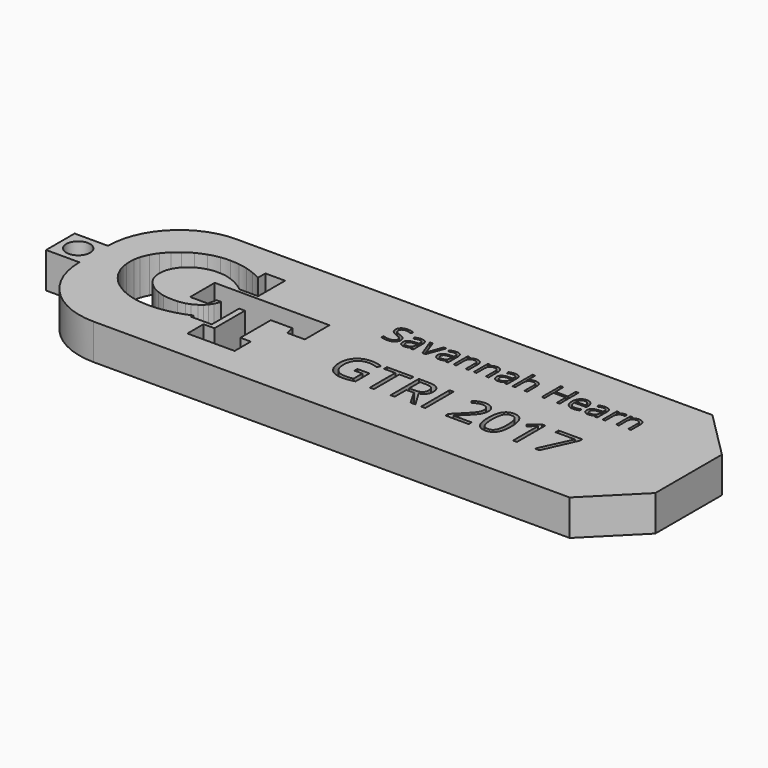
from build123d import *

# Parameters (mm, degrees)
F0_W         = 63.5
F0_H         = 19.05
F1_DEPTH     = 3.81
F3_DEPTH     = 3.81
F4_SIZE      = 5.08
F5_SIZE      = 5.08
F6_R         = 7.62
F7_R         = 7.62
F8_TEXT_SIZE = 3.5277777778
F10_DEPTH    = 1.524
F9_TEXT_SIZE = 5.2916666667
F11_DEPTH    = 1.524
F12_W        = 3.81
F12_H        = 3.81
F13_DEPTH    = 3.556
F15_D        = 2.54


# Not quite as in the source:
# - Text() gives the source's letters only with a copy of the font that has no kerning and outlines rounded to 1/6400 em; it was checked with that copy


with BuildPart() as f1:
    # F0 (on Top) → F1 (new body)
    with BuildSketch(Plane.XY):
        with Locations((31.75, -38.8746707218)):
            Rectangle(F0_W, F0_H)
    extrude(amount=F1_DEPTH)

    # F2 (on face) → F3 (cut)
    with BuildSketch(Plane.XY.offset(3.81)):
        with BuildLine():
            ThreePointArc((9.6262898296, -32.6765216887), (9.1345656228, -32.6782186949), (8.6470656097, -32.7425561845))
            ThreePointArc((8.6470656097, -32.7425561845), (8.0416604213, -32.8459942993), (7.4538225308, -33.0239310861))
            ThreePointArc((7.4538225308, -33.0239310861), (6.9355950201, -33.2250870831), (6.4325318672, -33.4616266191))
            ThreePointArc((6.4325318672, -33.4616266191), (5.9624118467, -33.7301717613), (5.5258763023, -34.0504311025))
            ThreePointArc((5.5258763023, -34.0504311025), (5.1852816432, -34.3165591196), (4.8669776879, -34.6089825034))
            ThreePointArc((4.8669776879, -34.6089825034), (4.5097063038, -34.9592664571), (4.1853138246, -35.3402011096))
            ThreePointArc((4.1853138246, -35.3402011096), (3.942059585, -35.6919738597), (3.7296244409, -36.0631719232))
            ThreePointArc((3.7296244409, -36.0631719232), (3.531707517, -36.4810877637), (3.3790939488, -36.9175896049))
            ThreePointArc((3.3790939488, -36.9175896049), (3.2938530275, -37.2302091826), (3.2438719645, -37.5503636897))
            ThreePointArc((3.2438719645, -37.5503636897), (3.2157331662, -38.0625072867), (3.2438719645, -38.5746508837))
            ThreePointArc((3.2438719645, -38.5746508837), (3.2872944597, -38.8672702316), (3.3429092728, -39.1578190029))
            ThreePointArc((3.3429092728, -39.1578190029), (3.3975529318, -39.3800627955), (3.4688711166, -39.597529918))
            ThreePointArc((3.4688711166, -39.597529918), (3.5952100841, -39.8924262154), (3.7296244409, -40.1837304235))
            ThreePointArc((3.7296244409, -40.1837304235), (3.8898334232, -40.4674932421), (4.0712854825, -40.7381653786))
            ThreePointArc((4.0712854825, -40.7381653786), (4.2164038702, -40.9343188623), (4.3698656373, -41.1240160465))
            ThreePointArc((4.3698656373, -41.1240160465), (4.4748950547, -41.2464015486), (4.5850998722, -41.3641482592))
            ThreePointArc((4.5850998722, -41.3641482592), (4.7484852476, -41.5319231994), (4.9246759154, -41.6861958802))
            ThreePointArc((4.9246759154, -41.6861958802), (5.085215868, -41.8163599874), (5.2489168011, -41.942525655))
            ThreePointArc((5.2489168011, -41.942525655), (5.3654646363, -42.0288014147), (5.4855244234, -42.110119015))
            ThreePointArc((5.4855244234, -42.110119015), (5.6214336133, -42.2028707503), (5.7604718022, -42.2908626497))
            ThreePointArc((5.7604718022, -42.2908626497), (5.8741145853, -42.3605784939), (5.9905075468, -42.4255989492))
            ThreePointArc((5.9905075468, -42.4255989492), (6.2169238827, -42.5464367765), (6.4516742714, -42.6501594484))
            ThreePointArc((6.4516742714, -42.6501594484), (6.7163385506, -42.7569305989), (6.9818515331, -42.8615733981))
            ThreePointArc((6.9818515331, -42.8615733981), (7.2850539518, -42.9552044529), (7.5919940136, -43.0357418954))
            ThreePointArc((7.5919940136, -43.0357418954), (7.8773558884, -43.0981583545), (8.1659872085, -43.143093586))
            ThreePointArc((8.1659872085, -43.143093586), (8.452848009, -43.1793154443), (8.7410761043, -43.2022437453))
            ThreePointArc((8.7410761043, -43.2022437453), (9.2430550429, -43.2262039196), (9.7455643117, -43.2197712362))
            ThreePointArc((9.7455643117, -43.2197712362), (10.2175816844, -43.1877010221), (10.6885796413, -43.143093586))
            ThreePointArc((10.6885796413, -43.143093586), (11.0944028016, -43.0662362996), (11.4988386631, -42.9823845625))
            ThreePointArc((11.4988386631, -42.9823845625), (11.7703194323, -42.9127287999), (12.0407473296, -42.8390912712))
            ThreePointArc((12.0407473296, -42.8390912712), (12.5181599326, -42.6898390275), (12.9890888929, -42.5212420523))
            ThreePointArc((12.9890888929, -42.5212420523), (13.1979634187, -42.4355467595), (13.4007316083, -42.3362627625))
            Line((13.4007316083, -42.3362627625), (13.4007316083, -42.6436923444))
            Line((13.4007316083, -42.6436923444), (15.6152648851, -42.6436923444))
            Line((15.6152648851, -42.6436923444), (15.6152648851, -38.9835685492))
            Line((15.6152648851, -38.9835685492), (16.2266530097, -38.9835685492))
            Line((16.2266530097, -38.9835685492), (16.2266530097, -43.0431254208))
            Line((16.2266530097, -43.0431254208), (15.0589663535, -43.0431254208))
            Line((15.0589663535, -43.0431254208), (15.0589663535, -45.1925210655))
            Line((15.0589663535, -45.1925210655), (20.0976803899, -45.1925210655))
            Line((20.0976803899, -45.1925210655), (20.0976803899, -43.0322438478))
            Line((20.0976803899, -43.0322438478), (18.9852751791, -43.0322438478))
            Line((18.9852751791, -43.0322438478), (18.9852751791, -38.9734357595))
            Line((18.9852751791, -38.9734357595), (21.3031545281, -38.9734357595))
            Line((21.3031545281, -38.9734357595), (21.4784201235, -39.9154871702))
            Line((21.4784201235, -39.9154871702), (23.3669020236, -39.9154871702))
            Line((23.3669020236, -39.9154871702), (23.3669020236, -36.6271026433))
            Line((23.3669020236, -36.6271026433), (11.1224930733, -36.6271026433))
            Line((11.1224930733, -36.6271026433), (11.1224930733, -39.9040654302))
            Line((11.1224930733, -39.9040654302), (13.0066871643, -39.9040654302))
            Line((13.0066871643, -39.9040654302), (13.1801906973, -38.9807745814))
            Line((13.1801906973, -38.9807745814), (13.6883091182, -38.9807745814))
            ThreePointArc((13.6883091182, -38.9807745814), (13.5726204471, -39.3085025724), (13.4228430688, -39.6221205592))
            ThreePointArc((13.4228430688, -39.6221205592), (13.2923973725, -39.8169791611), (13.1597043946, -40.0103144348))
            ThreePointArc((13.1597043946, -40.0103144348), (13.0200234247, -40.1756392664), (12.864947319, -40.3266176581))
            ThreePointArc((12.864947319, -40.3266176581), (12.6867217698, -40.4726760467), (12.4962525442, -40.602363646))
            ThreePointArc((12.4962525442, -40.602363646), (12.2400840685, -40.7479520063), (11.9757410139, -40.8781096339))
            ThreePointArc((11.9757410139, -40.8781096339), (11.7468865269, -40.9657469786), (11.5140965208, -41.0423204303))
            ThreePointArc((11.5140965208, -41.0423204303), (11.1541789739, -41.1217650759), (10.7890991494, -41.1724485457))
            ThreePointArc((10.7890991494, -41.1724485457), (10.0187817768, -41.1692547257), (9.25235264, -41.091889143))
            ThreePointArc((9.25235264, -41.091889143), (8.8774229201, -40.9918755502), (8.5149621591, -40.8533215523))
            ThreePointArc((8.5149621591, -40.8533215523), (8.2073861762, -40.72412104), (7.9107973725, -40.5713766813))
            ThreePointArc((7.9107973725, -40.5713766813), (7.6137187512, -40.3703173707), (7.3407134041, -40.1376187801))
            ThreePointArc((7.3407134041, -40.1376187801), (7.1064939389, -39.9085854316), (6.9038560614, -39.6511889994))
            ThreePointArc((6.9038560614, -39.6511889994), (6.7192820205, -39.3432356568), (6.5785367042, -39.0129424632))
            Line((6.5785367042, -39.0129424632), (6.5767983906, -39.0094779432))
            ThreePointArc((6.5767983906, -39.0094779432), (6.5492423445, -38.9362341195), (6.5244646942, -38.8620043316))
            ThreePointArc((6.5244646942, -38.8620043316), (6.4414726786, -38.230977645), (6.4979814924, -37.5970304012))
            ThreePointArc((6.4979814924, -37.5970304012), (6.5898893649, -37.2523307931), (6.7299287766, -36.9242243469))
            ThreePointArc((6.7299287766, -36.9242243469), (6.9113454374, -36.6120556231), (7.1233338676, -36.3197848201))
            ThreePointArc((7.1233338676, -36.3197848201), (7.4279401894, -36.0096111003), (7.7616400085, -35.7309766114))
            ThreePointArc((7.7616400085, -35.7309766114), (8.1219806737, -35.4885660649), (8.5149621591, -35.3037044406))
            ThreePointArc((8.5149621591, -35.3037044406), (8.8943731278, -35.1613795105), (9.2883650213, -35.0666195154))
            ThreePointArc((9.2883650213, -35.0666195154), (9.6384633606, -34.9957907429), (9.9952891469, -34.9796377122))
            ThreePointArc((9.9952891469, -34.9796377122), (10.3925075526, -34.988499992), (10.7890991494, -35.0125022233))
            ThreePointArc((10.7890991494, -35.0125022233), (11.1337253073, -35.071517669), (11.4696575329, -35.1684689522))
            ThreePointArc((11.4696575329, -35.1684689522), (11.7934513027, -35.2736863983), (12.102752924, -35.4159735143))
            ThreePointArc((12.102752924, -35.4159735143), (12.4102322735, -35.5683354788), (12.7124004066, -35.7309766114))
            ThreePointArc((12.7124004066, -35.7309766114), (12.9426050459, -35.8697422563), (13.1597043946, -36.0282287002))
            ThreePointArc((13.1597043946, -36.0282287002), (13.295231463, -36.1369667627), (13.4228430688, -36.2548939884))
            Line((13.4228430688, -36.2548939884), (15.4634509236, -36.2548939884))
            Line((15.4634509236, -36.2548939884), (15.4634509236, -32.6641239226))
            Line((15.4634509236, -32.6641239226), (13.3566195145, -32.6641239226))
            Line((13.3566195145, -32.6641239226), (13.3566195145, -33.6617715657))
            ThreePointArc((13.3566195145, -33.6617715657), (12.8964143847, -33.4146596901), (12.4085452408, -33.2280136645))
            ThreePointArc((12.4085452408, -33.2280136645), (11.9788401114, -33.0582867127), (11.5348305553, -32.9305790365))
            ThreePointArc((11.5348305553, -32.9305790365), (11.0856293232, -32.8129183237), (10.6239356101, -32.7632725239))
            ThreePointArc((10.6239356101, -32.7632725239), (10.1280029956, -32.6866585625), (9.6262898296, -32.6765216887))
        make_face()
    extrude(amount=-F3_DEPTH, mode=Mode.SUBTRACT)

    # F4
    f4_edges = [f1.edges().sort_by_distance(p)[0] for p in [
        (63.5, -48.399671, 1.905),
    ]]
    chamfer(f4_edges, length=F4_SIZE)

    # F5
    f5_edges = [f1.edges().sort_by_distance(p)[0] for p in [
        (63.5, -29.349671, 1.905),
    ]]
    chamfer(f5_edges, length=F5_SIZE)

    # F6
    f6_edges = [f1.edges().sort_by_distance(p)[0] for p in [
        (0, -48.399671, 1.905),
    ]]
    fillet(f6_edges, radius=F6_R)

    # F7
    f7_edges = [f1.edges().sort_by_distance(p)[0] for p in [
        (0, -29.349671, 1.905),
    ]]
    fillet(f7_edges, radius=F7_R)

    # F8 (on face) → F10 (cut)
    with BuildSketch(Plane.XY.offset(3.81)):
        with Locations((27.94, -35.6996707218)):
            Text('Savannah Hearn', F8_TEXT_SIZE, font='Open Sans', text_align=(TextAlign.LEFT, TextAlign.BOTTOM))
    extrude(amount=-F10_DEPTH, mode=Mode.SUBTRACT)

    # F9 (on face) → F11 (cut)
    with BuildSketch(Plane.XY.offset(3.81)):
        with Locations((27.94, -43.3196707218)):
            Text('GTRI 2017', F9_TEXT_SIZE, font='Open Sans', text_align=(TextAlign.LEFT, TextAlign.BOTTOM))
    extrude(amount=-F11_DEPTH, mode=Mode.SUBTRACT)

    # F12 (on face) → F13 (join)
    with BuildSketch(Plane(origin=(0, 0, 0), x_dir=(0, -1, 0), z_dir=(-1, 0, 0))):
        with Locations((38.8746707218, 1.905)):
            Rectangle(F12_W, F12_H)
    extrude(amount=F13_DEPTH)

    # F15 (through all)
    with Locations(Plane.XY.offset(3.81)):
        with Locations((-1.651, -38.8746707218)):
            Hole(F15_D / 2)


solid = f1.part
